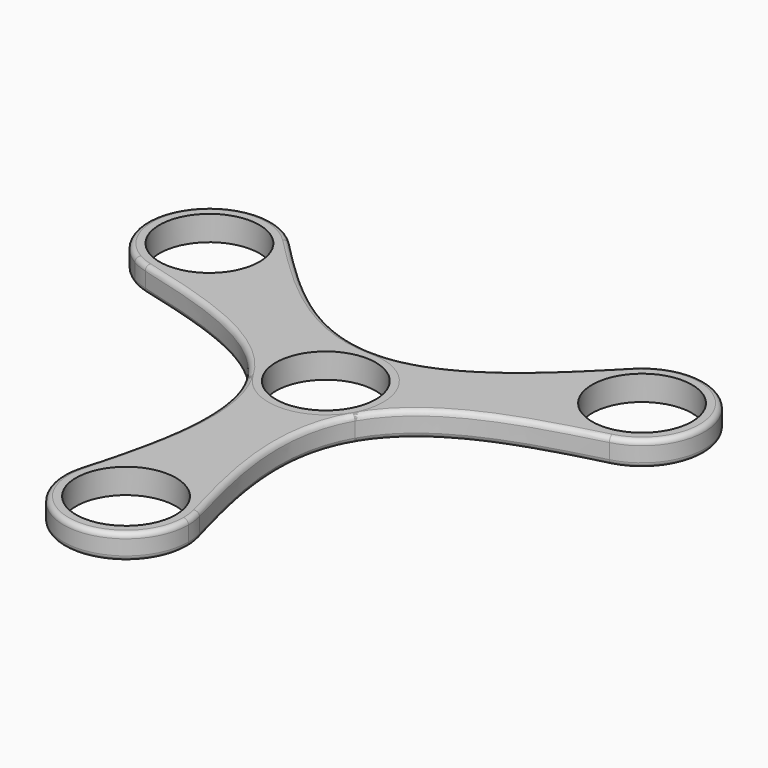
from build123d import *

# Parameters (mm, degrees)
F0_R     = 5.08
F1_DEPTH = 2.54
F2_R     = 0.508
F4_COUNT = 3


# Not quite as in the source:
# - a feature names something its author has since deleted; it is built from what else it names


with BuildPart() as f1:
    # F0 (on Top) → F1 (new body)
    with BuildSketch(Plane.XY):
        with BuildLine():
            ThreePointArc((5.4967904929, -3.1792757472), (6.132989468, -1.6458858359), (6.35, 0))
            ThreePointArc((6.35, 0), (-1.6458858359, 6.132989468), (-5.4967904929, -3.1792757472))
            ThreePointArc((-5.4967904929, -3.1792757472), (0, -6.35), (5.4967904929, -3.1792757472))
        make_face()
        Circle(F0_R, mode=Mode.SUBTRACT)
        with BuildLine():
            ThreePointArc((5.4967904929, -3.1792757472), (0, -6.35), (-5.4967904929, -3.1792757472))
            add(Edge.make_bspline(
                [(-5.4967904929, -3.1792757472), (-2.1172126289, -9.0223774314), (-4.238916561, -16.8614275753), (-6.1229987764, -23.7173277254)],
                knots=[0, 0, 0, 0, 20.5475963527, 20.5475963527, 20.5475963527, 20.5475963527], degree=3))
            ThreePointArc((-6.1229987764, -23.7173277254), (0, -19.05), (6.1229987764, -23.7173277254))
            add(Edge.make_bspline(
                [(5.4967904929, -3.1792757472), (2.1172126289, -9.0223774314), (4.238916561, -16.8614275753), (6.1229987764, -23.7173277254)],
                knots=[0, 0, 0, 0, 20.5475963527, 20.5475963527, 20.5475963527, 20.5475963527], degree=3))
        make_face()
        with BuildLine():
            ThreePointArc((6.1229987764, -23.7173277254), (0, -19.05), (-6.1229987764, -23.7173277254))
            ThreePointArc((-6.1229987764, -23.7173277254), (-0.8489575283, -31.6929938118), (6.35, -25.4))
            ThreePointArc((6.35, -25.4), (6.2929938118, -24.5510424717), (6.1229987764, -23.7173277254))
        make_face()
        with Locations((0, -25.4)):
            Circle(F0_R, mode=Mode.SUBTRACT)
    extrude(amount=F1_DEPTH)

    # F2
    f2_edges = [f1.edges().sort_by_distance(p)[0] for p in [
        (0, 6.35, 2.54),
        (0, -31.75, 2.54),
        (0, -31.75, 0),
        (0, 6.35, 0),
    ]]
    fillet(f2_edges, radius=F2_R)


with BuildPart() as f4_1:
    # F4: instance of F1
    add(f1.part.rotate(Axis((0, 0, 8.1363003701), (0, 0, 1)), 1 * 360 / F4_COUNT))


with BuildPart() as f4_2:
    # F4: instance of F1
    add(f1.part.rotate(Axis((0, 0, 8.1363003701), (0, 0, 1)), 2 * 360 / F4_COUNT))


solid = Compound([f1.part, f4_1.part, f4_2.part])
